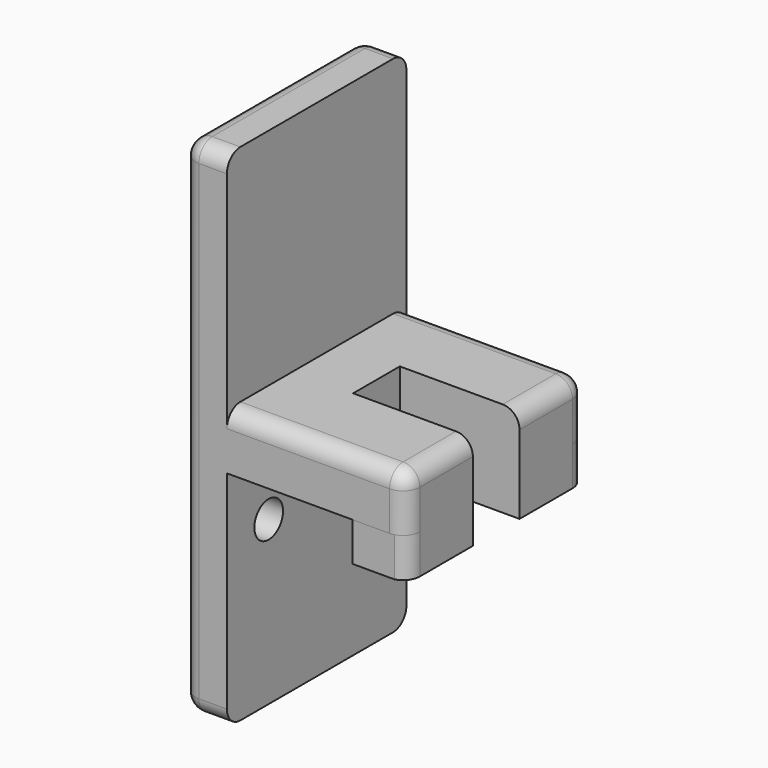
from build123d import *

# Parameters (mm, degrees)
F0_W     = 20
F0_H     = 5
F0_W_2   = 10
F0_H_2   = 3.8665379398
F0_H_3   = 20
F0_R     = 1.6
F1_DEPTH = 4
F2_DEPTH = 20
F3_DEPTH = 66
F4_R     = 1.5
F6_DEPTH = 3.5
F7_DEPTH = 3.5
F8_DEPTH = 25


# Not quite as in the source:
# - an extrude ends at something that could not be found from the text; its depth is read off the source's solid


with BuildPart() as f1:
    # F0 (on Right) → F1 (new body)
    with BuildSketch(Plane.YZ):
        Polygon((3.6049238205, -6.8721993268), (3.6049238205, 13.1278006732), (-16.3950761795, 13.1278006732), (-16.3950761795, 6.6331364214), (-6.3950761795, 6.6331364214), (-6.3950761795, 2.7665984817), (-16.3950761795, 2.7665984817), (-16.3950761795, -6.8721993268), align=None)
        with Locations((-6.3950761795, -9.3721993268)):
            Rectangle(F0_W, F0_H)
        with Locations((-11.3950761795, 4.6998674516)):
            Rectangle(F0_W_2, F0_H_2)
        with Locations((-6.3950761795, -21.8721993268)):
            Rectangle(F0_W, F0_H_3)
        with Locations((-11.7450761795, -17.3721993268)):
            Circle(F0_R, mode=Mode.SUBTRACT)
        with Locations((-1.0450761795, -17.3721993268)):
            Circle(F0_R, mode=Mode.SUBTRACT)
    extrude(amount=F1_DEPTH)

    # F0 (on Right) → F2 (join)
    with BuildSketch(Plane.YZ):
        with Locations((-6.3950761795, -9.3721993268)):
            Rectangle(F0_W, F0_H)
    extrude(amount=F2_DEPTH)

    # F0 (on Right) → F3 (cut, through all)
    with BuildSketch(Plane.YZ):
        with Locations((-1.0450761795, -17.3721993268)):
            Circle(F0_R)
    extrude(amount=-F3_DEPTH, mode=Mode.SUBTRACT)

    # F4
    f4_edges = [f1.edges().sort_by_distance(p)[0] for p in [
        (0, 3.604924, -9.372199),
        (0, -6.395076, 13.127801),
        (0, -16.395076, -9.372199),
        (0, -6.395076, -31.872199),
        (2, 3.604924, 13.127801),
        (2, 3.604924, -31.872199),
        (2, -16.395076, 13.127801),
        (2, -16.395076, -31.872199),
        (12, -16.395076, -6.872199),
        (12, 3.604924, -6.872199),
        (20, -6.395076, -6.872199),
        (20, 3.604924, -9.372199),
        (20, -16.395076, -9.372199),
    ]]
    fillet(f4_edges, radius=F4_R)

    # F5 (on face) → F6 (join)
    with BuildSketch(Plane(origin=(0, 0, -11.8721993268), x_dir=(1, 0, 0), z_dir=(0, 0, -1))):
        with BuildLine():
            Line((15.1547100395, 8.9950761795), (20, 8.9950761795))
            Line((20, 8.9950761795), (20, 14.8950761795))
            ThreePointArc((20, 14.8950761795), (19.686066448, 15.8133606567), (18.8756714919, 16.3472713903))
            Line((18.8756714919, 16.3472713903), (15.1547100395, 16.3472713903))
            Line((15.1547100395, 16.3472713903), (15.1547100395, 8.9950761795))
        make_face()
        with BuildLine():
            Line((20, -2.1049238205), (20, 3.7950761795))
            Line((20, 3.7950761795), (15.1547100395, 3.7950761795))
            Line((15.1547100395, 3.7950761795), (15.1547100395, -3.5571190313))
            Line((15.1547100395, -3.5571190313), (18.8756714919, -3.5571190313))
            ThreePointArc((18.8756714919, -3.5571190313), (19.686066448, -3.0232082977), (20, -2.1049238205))
        make_face()
    extrude(amount=F6_DEPTH)

    # F5 (on face) → F7 (join)
    with BuildSketch(Plane(origin=(0, 0, -11.8721993268), x_dir=(1, 0, 0), z_dir=(0, 0, -1))):
        with BuildLine():
            Line((15.1547100395, 8.9950761795), (20, 8.9950761795))
            Line((20, 8.9950761795), (20, 14.8950761795))
            ThreePointArc((20, 14.8950761795), (19.686066448, 15.8133606567), (18.8756714919, 16.3472713903))
            Line((18.8756714919, 16.3472713903), (15.1547100395, 16.3472713903))
            Line((15.1547100395, 16.3472713903), (15.1547100395, 8.9950761795))
        make_face()
    extrude(amount=F7_DEPTH)

    # F5 (on face) → F8 (cut)
    with BuildSketch(Plane(origin=(0, 0, -11.8721993268), x_dir=(1, 0, 0), z_dir=(0, 0, -1))):
        Polygon((20, 3.7950761795), (20, 8.9950761795), (15.1547100395, 8.9950761795), (9.3279955909, 8.9950761795), (9.3279955909, 3.7950761795), (15.1547100395, 3.7950761795), align=None)
    extrude(amount=-F8_DEPTH, mode=Mode.SUBTRACT)


solid = f1.part
